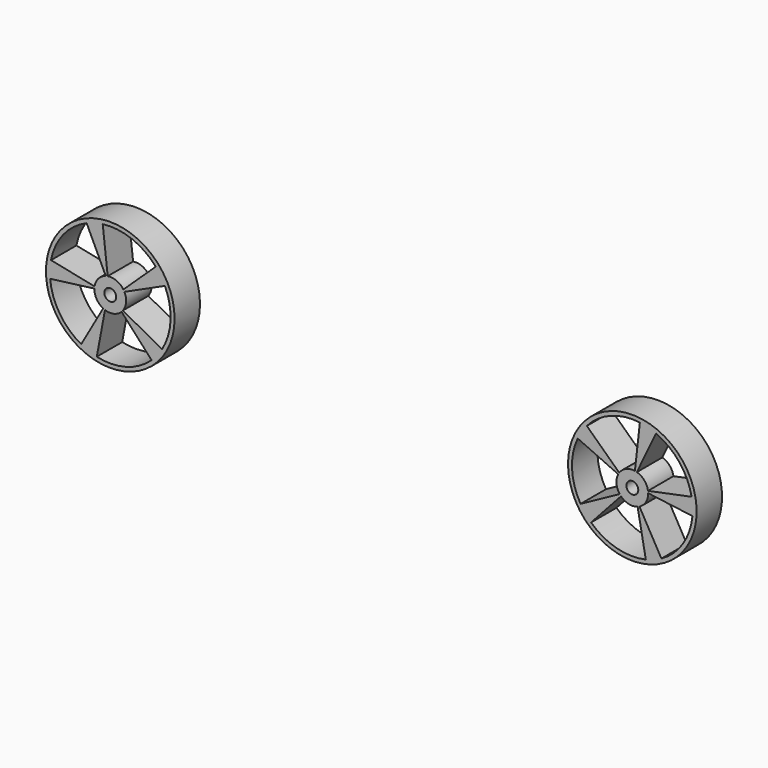
from build123d import *

# Parameters (mm, degrees)
F0_R            = 162
F0_R_2          = 15
F1_DEPTH        = 40
F1_COPIES_COUNT = 5


# Not quite as in the source:
# - a pattern or mirror of a feature is missing from the dataset's text; its kind, count and spacing are read off the source's solid
# - a feature names something its author has since deleted; it is built from what else it names


with BuildPart() as f1:
    # F0 (on Front) → F1 (new body, symmetric)
    with BuildSketch(Plane.XZ):
        with Locations((-657.5, 0)):
            Circle(F0_R)
        with BuildLine():
            ThreePointArc((-676.4987085863, 150.8079874279), (-556.9609620722, 113.9995695279), (-505.5, 0))
            ThreePointArc((-505.5, 0), (-741.3053398481, -126.8095619933), (-717.0876975387, 139.8331373532))
            ThreePointArc((-717.0876975387, 139.8331373532), (-697.1745213008, 146.7308159847), (-676.4987085863, 150.8079874279))
        make_face(mode=Mode.SUBTRACT)
        with BuildLine():
            ThreePointArc((-617.5, 0), (-631.618859249, 30.4986319927), (-664.0083276714, 39.4669693658))
            ThreePointArc((-664.0083276714, 39.4669693658), (-666.472603334, 38.9806668672), (-668.9014980889, 38.3406552021))
            ThreePointArc((-668.9014980889, 38.3406552021), (-681.4158950956, -32.0629063214), (-617.5, 0))
        make_face()
        with Locations((-657.5, 0)):
            Circle(F0_R_2, mode=Mode.SUBTRACT)
        with BuildLine():
            Line((-664.0083276714, 39.4669693658), (-676.4987085863, 150.8079874279))
            ThreePointArc((-676.4987085863, 150.8079874279), (-697.1745213008, 146.7308159847), (-717.0876975387, 139.8331373532))
            Line((-717.0876975387, 139.8331373532), (-668.9014980889, 38.3406552021))
            ThreePointArc((-668.9014980889, 38.3406552021), (-666.472603334, 38.9806668672), (-664.0083276714, 39.4669693658))
        make_face()
    extrude(amount=F1_DEPTH, both=True)

    # F1_copies: F1 ×5 about axis
    f1_copies_axis = Axis((-657.5, 0, 0), (0, 1, 0))


with BuildPart() as f1_1:
    add(f1.part)
    for i in range(1, F1_COPIES_COUNT):
        add(f1.part.rotate(f1_copies_axis, i * 360 / F1_COPIES_COUNT))


with BuildPart() as f2_1:
    # F2: instance of F1
    add(f1_1.part.mirror(Plane.YZ))


solid = Compound([f1_1.part, f2_1.part])
